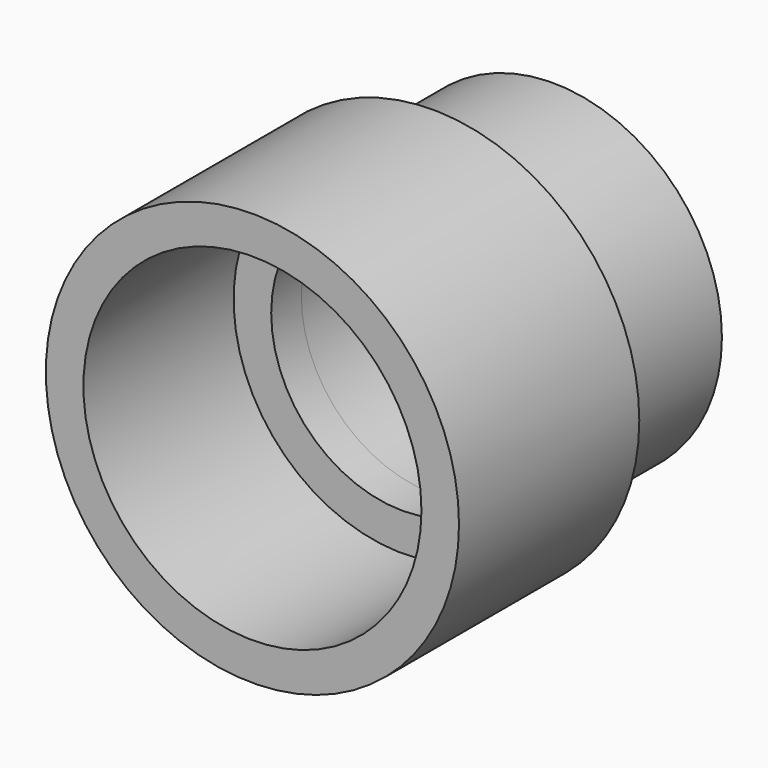
from build123d import *

# Parameters (mm, degrees)
F0_R          = 11
F0_R_2        = 9
F1_DEPTH      = 12
F0_R_3        = 7
F2_DEPTH      = 8
F2_DEPTH_BACK = 2


# Not quite as in the source:
# - a feature names something its author has since deleted; it is built from what else it names


with BuildPart() as f1:
    # F0 (on Front) → F1 (new body)
    with BuildSketch(Plane.XZ):
        Circle(F0_R)
        Circle(F0_R_2, mode=Mode.SUBTRACT)
    extrude(amount=F1_DEPTH)


with BuildPart() as f2:
    # F0 (on Front) → F2 (new body, two sides)
    with BuildSketch(Plane.XZ) as f2_sk:
        Circle(F0_R_2)
        Circle(F0_R_3, mode=Mode.SUBTRACT)
    extrude(amount=-F2_DEPTH)
    extrude(f2_sk.sketch, amount=F2_DEPTH_BACK)


solid = Compound([f1.part, f2.part])
